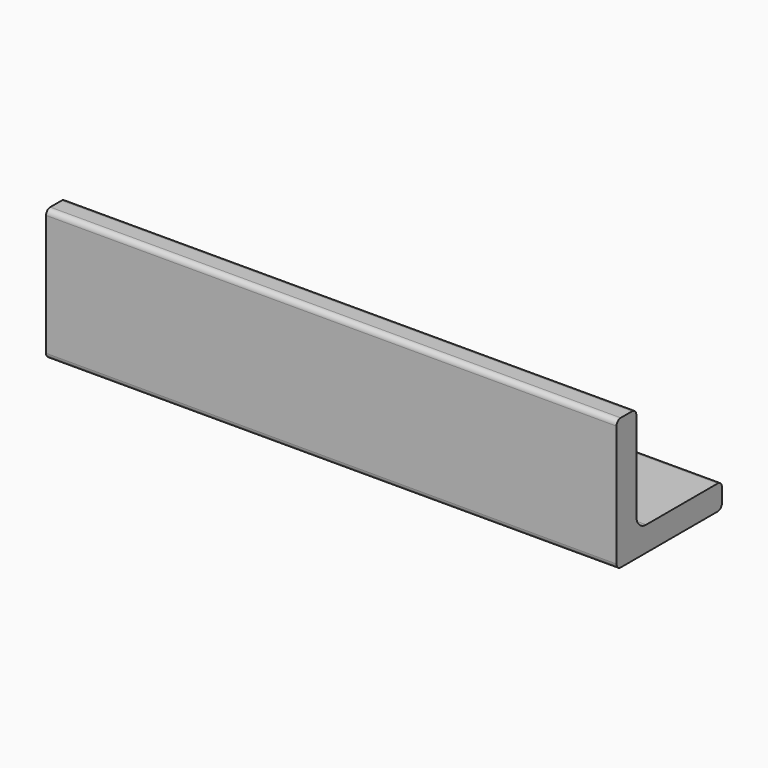
from build123d import *

# Parameters (mm, degrees)
F1_DEPTH = 55
F2_R     = 1
F3_R     = 2.38125
F4_R     = 3.25
F5_DEPTH = 25
F6_SIZE  = 0.5


with BuildPart() as f1:
    # F0 (on Right) → F1 (new body, symmetric)
    with BuildSketch(Plane.YZ):
        Polygon((0, 25.4), (0, 0), (25.4, 0), (25.4, 4.7625), (4.7625, 4.7625), (4.7625, 25.4), align=None)
    extrude(amount=F1_DEPTH, both=True)

    # F2
    f2_edges = [f1.edges().sort_by_distance(p)[0] for p in [
        (0, 0, 25.4),
        (0, 4.7625, 25.4),
        (0, 0, 0),
        (0, 25.4, 4.7625),
        (0, 25.4, 0),
    ]]
    fillet(f2_edges, radius=F2_R)

    # F3
    f3_edges = [f1.edges().sort_by_distance(p)[0] for p in [
        (0, 4.7625, 4.7625),
    ]]
    fillet(f3_edges, radius=F3_R)

    # F4 (on face) → F5 (cut)
    with BuildSketch(Plane.XY.offset(4.7625)):
        with Locations((-40, 15)):
            Circle(F4_R)
        with Locations((690, 15)):
            Circle(F4_R)
        with Locations((1420, 15)):
            Circle(F4_R)
        with Locations((40, 15)):
            Circle(F4_R)
    extrude(amount=-F5_DEPTH, mode=Mode.SUBTRACT)

    # F6
    f6_edges = [f1.edges().sort_by_distance(p)[0] for p in [
        (-43.25, 15, 4.7625),
        (-36.75, 15, 2.38125),
        (-43.25, 15, 0),
        (36.75, 15, 4.7625),
        (43.25, 15, 2.38125),
        (36.75, 15, 0),
    ]]
    chamfer(f6_edges, length=F6_SIZE)


solid = f1.part
